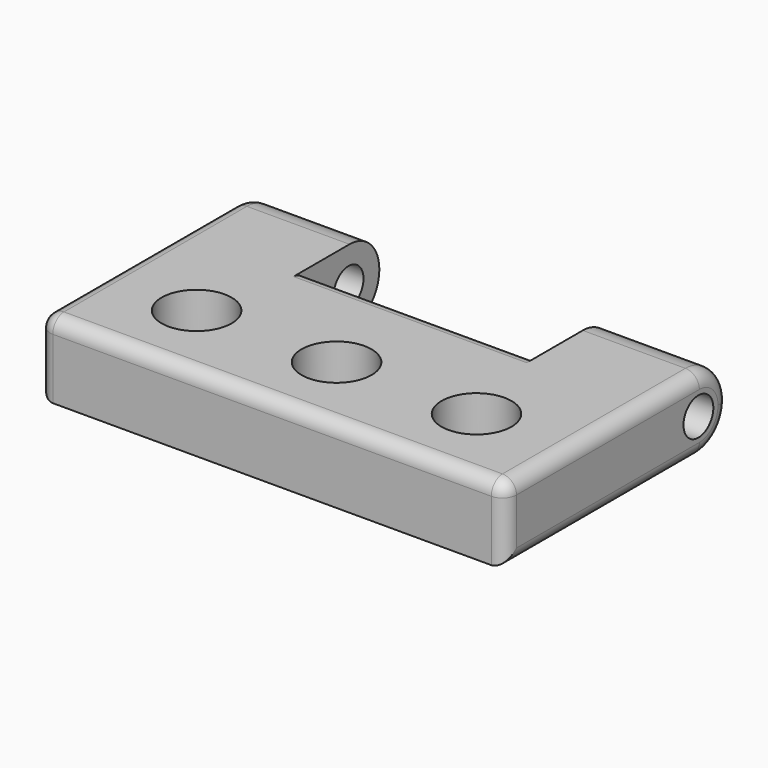
from build123d import *

# Parameters (mm, degrees)
F0_R     = 2
F1_DEPTH = 8
F2_R     = 2
F3_DEPTH = 60
F4_R     = 3.99999
F5_R     = 1.5
F6_R     = 3.75
F7_DEPTH = 6
F8_SIZE  = 1
F9_R     = 1.5


# Not quite as in the source:
# - a fillet or chamfer is up to 0.001 mm smaller than in the source, because OpenCascade refuses the exact size


with BuildPart() as f1:
    # F0 (on Top) → F1 (new body)
    with BuildSketch(Plane.XY):
        Polygon((25, -15), (25, 15), (12.5, 15), (12.5, 5), (-12.5, 5), (-12.5, 15), (-25, 15), (-25, -15), align=None)
        with Locations((-15, -6.3565024175)):
            Circle(F0_R, mode=Mode.SUBTRACT)
        with Locations((0, -6.3565024175)):
            Circle(F0_R, mode=Mode.SUBTRACT)
        with Locations((15, -6.3565024175)):
            Circle(F0_R, mode=Mode.SUBTRACT)
    extrude(amount=F1_DEPTH)

    # F2 (on face) → F3 (cut)
    with BuildSketch(Plane(origin=(-25, 0, 0), x_dir=(0, -1, 0), z_dir=(-1, 0, 0))):
        with Locations((-10.8748758212, 4)):
            Circle(F2_R)
    extrude(amount=-F3_DEPTH, mode=Mode.SUBTRACT)

    # F4 (radius 4 in the source; OpenCascade refuses exactly that, so slightly less here)
    f4_edges = [f1.edges().sort_by_distance(p)[0] for p in [
        (-18.75, 15, 8),
        (18.75, 15, 8),
        (-18.75, 15, 0),
        (18.75, 15, 0),
    ]]
    fillet(f4_edges, radius=F4_R)

    # F5
    f5_edges = [f1.edges().sort_by_distance(p)[0] for p in [
        (0, 5, 8),
        (0, -15, 8),
    ]]
    fillet(f5_edges, radius=F5_R)

    # F6 (on face) → F7 (cut)
    with BuildSketch(Plane.XY.offset(8)):
        with Locations((-15, -6.3565024175)):
            Circle(F6_R)
        with Locations((0, -6.3565024175)):
            Circle(F6_R)
        with Locations((15, -6.3565024175)):
            Circle(F6_R)
    extrude(amount=-F7_DEPTH, mode=Mode.SUBTRACT)

    # F8
    f8_edges = [f1.edges().sort_by_distance(p)[0] for p in [
        (-17, -6.356502, 2),
        (-2, -6.356502, 2),
        (13, -6.356502, 2),
    ]]
    chamfer(f8_edges, length=F8_SIZE)

    # F9
    f9_edges = [f1.edges().sort_by_distance(p)[0] for p in [
        (25, -1.249995, 8),
        (-25, -1.249995, 8),
    ]]
    fillet(f9_edges, radius=F9_R)


solid = f1.part
